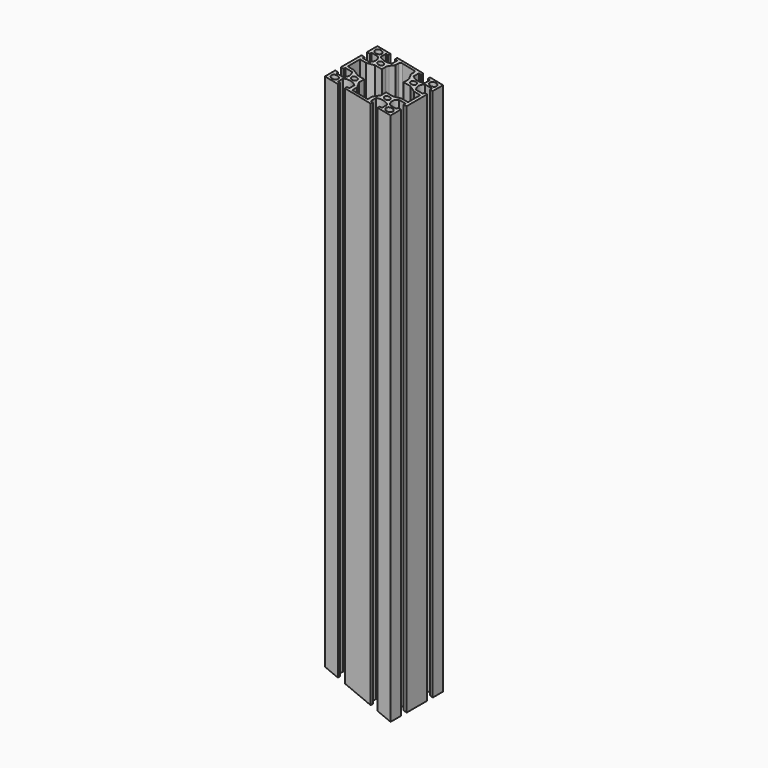
from build123d import *

# Parameters (mm, degrees)
F0_R          = 3
F0_R_2        = 2.5
F1_DEPTH      = 500
F2_R          = 2
F3_R          = 7
F6_DEPTH      = 30
F6_DEPTH_BACK = 30


# Not quite as in the source:
# - a feature names something its author has since deleted; it is built from what else it names


with BuildPart() as f1:
    # F0 (on Top) → F1 (new body)
    with BuildSketch(Plane.XY):
        with BuildLine():
            Line((18.15, -30), (30, -30))
            Line((30, -30), (30, -18.15))
            Line((30, -18.15), (27.5, -18.15))
            Line((27.5, -18.15), (27.5, -20.15))
            Line((27.5, -20.15), (21.5477069044, -20.15))
            ThreePointArc((21.5477069044, -20.15), (19.5, -15), (21.5477069044, -9.85))
            Line((21.5477069044, -9.85), (27.5, -9.85))
            Line((27.5, -9.85), (27.5, -11.85))
            Line((27.5, -11.85), (30, -11.85))
            Line((30, -11.85), (30, 11.85))
            Line((30, 11.85), (27.5, 11.85))
            Line((27.5, 11.85), (27.5, 9.85))
            Line((27.5, 9.85), (21.5477069044, 9.85))
            ThreePointArc((21.5477069044, 9.85), (19.5, 15), (21.5477069044, 20.15))
            Line((21.5477069044, 20.15), (27.5, 20.15))
            Line((27.5, 20.15), (27.5, 18.15))
            Line((27.5, 18.15), (30, 18.15))
            Line((30, 18.15), (30, 30))
            Line((30, 30), (18.15, 30))
            Line((18.15, 30), (18.15, 27.5))
            Line((18.15, 27.5), (20.15, 27.5))
            Line((20.15, 27.5), (20.15, 21.5477069044))
            ThreePointArc((20.15, 21.5477069044), (15, 19.5), (9.85, 21.5477069044))
            Line((9.85, 21.5477069044), (9.85, 27.5))
            Line((9.85, 27.5), (11.85, 27.5))
            Line((11.85, 27.5), (11.85, 30))
            Line((11.85, 30), (-11.85, 30))
            Line((-11.85, 30), (-11.85, 27.5))
            Line((-11.85, 27.5), (-9.85, 27.5))
            Line((-9.85, 27.5), (-9.85, 21.5477069044))
            ThreePointArc((-9.85, 21.5477069044), (-15, 19.5), (-20.15, 21.5477069044))
            Line((-20.15, 21.5477069044), (-20.15, 27.5))
            Line((-20.15, 27.5), (-18.15, 27.5))
            Line((-18.15, 27.5), (-18.15, 30))
            Line((-18.15, 30), (-30, 30))
            Line((-30, 30), (-30, 18.15))
            Line((-30, 18.15), (-27.5, 18.15))
            Line((-27.5, 18.15), (-27.5, 20.15))
            Line((-27.5, 20.15), (-21.5477069044, 20.15))
            ThreePointArc((-21.5477069044, 20.15), (-19.5, 15), (-21.5477069044, 9.85))
            Line((-21.5477069044, 9.85), (-27.5, 9.85))
            Line((-27.5, 9.85), (-27.5, 11.85))
            Line((-27.5, 11.85), (-30, 11.85))
            Line((-30, 11.85), (-30, -11.85))
            Line((-30, -11.85), (-27.5, -11.85))
            Line((-27.5, -11.85), (-27.5, -9.85))
            Line((-27.5, -9.85), (-21.5477069044, -9.85))
            ThreePointArc((-21.5477069044, -9.85), (-19.5, -15), (-21.5477069044, -20.15))
            Line((-21.5477069044, -20.15), (-27.5, -20.15))
            Line((-27.5, -20.15), (-27.5, -18.15))
            Line((-27.5, -18.15), (-30, -18.15))
            Line((-30, -18.15), (-30, -30))
            Line((-30, -30), (-18.15, -30))
            Line((-18.15, -30), (-18.15, -27.5))
            Line((-18.15, -27.5), (-20.15, -27.5))
            Line((-20.15, -27.5), (-20.15, -21.5477069044))
            ThreePointArc((-20.15, -21.5477069044), (-15, -19.5), (-9.85, -21.5477069044))
            Line((-9.85, -21.5477069044), (-9.85, -27.5))
            Line((-9.85, -27.5), (-11.85, -27.5))
            Line((-11.85, -27.5), (-11.85, -30))
            Line((-11.85, -30), (11.85, -30))
            Line((11.85, -30), (11.85, -27.5))
            Line((11.85, -27.5), (9.85, -27.5))
            Line((9.85, -27.5), (9.85, -21.5477069044))
            ThreePointArc((9.85, -21.5477069044), (15, -19.5), (20.15, -21.5477069044))
            Line((20.15, -21.5477069044), (20.15, -27.5))
            Line((20.15, -27.5), (18.15, -27.5))
            Line((18.15, -27.5), (18.15, -30))
        make_face()
        with Locations((-25, -25)):
            Circle(F0_R, mode=Mode.SUBTRACT)
        with Locations((-15, -15)):
            Circle(F0_R_2, mode=Mode.SUBTRACT)
        with Locations((25, -25)):
            Circle(F0_R, mode=Mode.SUBTRACT)
        with Locations((15, -15)):
            Circle(F0_R_2, mode=Mode.SUBTRACT)
        with Locations((-25, 25)):
            Circle(F0_R, mode=Mode.SUBTRACT)
        with Locations((-15, 15)):
            Circle(F0_R_2, mode=Mode.SUBTRACT)
        Polygon((-7, 22), (-7, 27.5), (0, 27.5), (7, 27.5), (7, 22), (10, 16), (10, 10), (16, 10), (22, 7), (27.5, 7), (27.5, 0), (27.5, -7), (22, -7), (16, -10), (10, -10), (10, -16), (7, -22), (7, -27.5), (0, -27.5), (-7, -27.5), (-7, -22), (-10, -16), (-10, -10), (-16, -10), (-22, -7), (-27.5, -7), (-27.5, 0), (-27.5, 7), (-22, 7), (-16, 10), (-10, 10), (-10, 16), align=None, mode=Mode.SUBTRACT)
        with Locations((15, 15)):
            Circle(F0_R_2, mode=Mode.SUBTRACT)
        with Locations((25, 25)):
            Circle(F0_R, mode=Mode.SUBTRACT)
    extrude(amount=F1_DEPTH)

    # F2
    f2_edges = [f1.edges().sort_by_distance(p)[0] for p in [
        (-7, 27.5, 250),
        (7, 27.5, 250),
    ]]
    fillet(f2_edges, radius=F2_R)

    # F3
    f3_edges = [f1.edges().sort_by_distance(p)[0] for p in [
        (-10, 16, 250),
        (10, 16, 250),
    ]]
    fillet(f3_edges, radius=F3_R)

    # F5 (on Front) → F6 (cut, two sides)
    with BuildSketch(Plane.XZ) as f6_sk:
        Polygon((190.5190290352, 666.216575566), (10.1971706169, 702.0848233142), (-30, 500), (150.3218584183, 464.1317522517), align=None)
        Polygon((-47.8999755124, -188.0671773906), (30, 0), (-147.6190188423, 73.5722065399), (-225.5189943547, -114.4949708507), align=None)
    extrude(amount=F6_DEPTH, mode=Mode.SUBTRACT)
    extrude(f6_sk.sketch, amount=-F6_DEPTH_BACK, mode=Mode.SUBTRACT)


solid = f1.part
